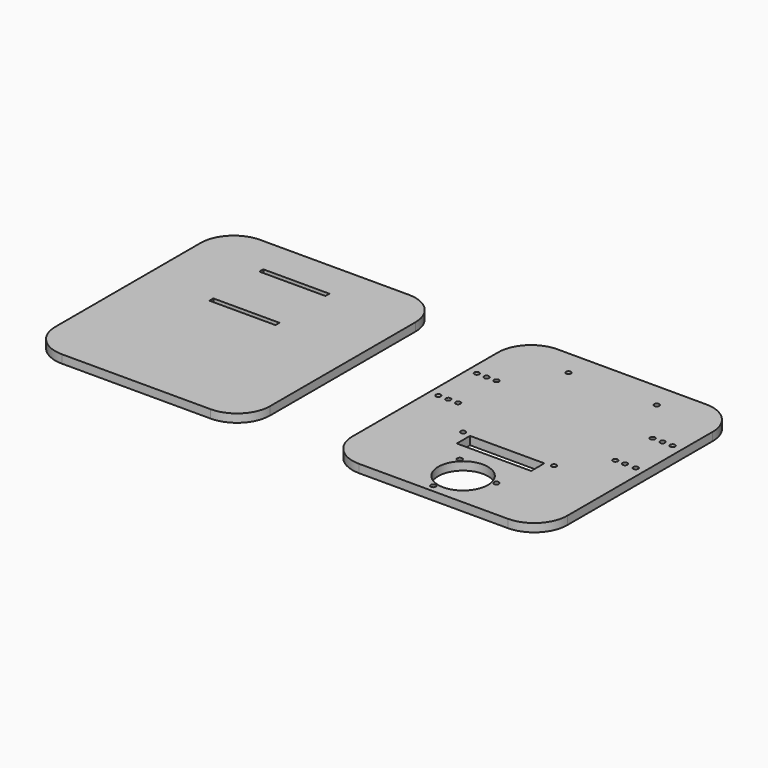
from build123d import *

# Parameters (mm, degrees)
F0_R     = 1.5000012089
F0_R_2   = 15.0000120892
F0_W     = 63
F0_H     = 28
F0_R_3   = 1.5
F0_W_2   = 45
F0_H_2   = 10
F1_DEPTH = 5
F0_W_3   = 40
F0_H_3   = 3
F2_DEPTH = 5


# Not quite as in the source:
# - a feature names something its author has since deleted; it is built from what else it names


with BuildPart() as f1:
    # F0 (on Top) → F1 (new body)
    with BuildSketch(Plane.XY):
        with BuildLine():
            Line((109.2777046029, -4.8284545538), (19.2777046029, -4.7197510892))
            ThreePointArc((19.2777046029, -4.7197510892), (5.1199557962, -10.5690629101), (-0.746451705, -24.719736501))
            Line((-0.746451705, -24.719736501), (-0.746451705, -134.8525817028))
            ThreePointArc((-0.746451705, -134.8525817028), (5.1114126713, -148.9947173266), (19.253548295, -154.8525817028))
            Line((19.253548295, -154.8525817028), (109.253548295, -154.8525817028))
            ThreePointArc((109.253548295, -154.8525817028), (123.3956839188, -148.9947173266), (129.253548295, -134.8525817028))
            Line((129.253548295, -134.8525817028), (129.253548295, -24.8284399656))
            ThreePointArc((129.253548295, -24.8284399656), (123.404221886, -10.6948474668), (109.2777046029, -4.8284545538))
        make_face()
        with Locations((60.6492295242, -150.5000877334)):
            Circle(F0_R, mode=Mode.SUBTRACT)
        with Locations((65.3296712528, -133.7744518814)):
            Circle(F0_R_2, mode=Mode.SUBTRACT)
        with Locations((82.2305977345, -129.661552608)):
            Circle(F0_R, mode=Mode.SUBTRACT)
        with Locations((53.3932128331, -121.3908070522)):
            Circle(F0_R, mode=Mode.SUBTRACT)
        with Locations((64.7868365049, -98.7337777073)):
            Rectangle(F0_W, F0_H, mode=Mode.SUBTRACT)
        with Locations((4.8244629152, -76.8351420979)):
            Circle(F0_R, mode=Mode.SUBTRACT)
        with Locations((10.8244677509, -76.8464319149)):
            Circle(F0_R, mode=Mode.SUBTRACT)
        with Locations((16.8244725865, -76.8634664953)):
            Circle(F0_R, mode=Mode.SUBTRACT)
        with Locations((4.8244629152, -47.7516189505)):
            Circle(F0_R, mode=Mode.SUBTRACT)
        with Locations((10.8244677509, -47.8464085426)):
            Circle(F0_R, mode=Mode.SUBTRACT)
        with Locations((16.8244725865, -47.8634431229)):
            Circle(F0_R, mode=Mode.SUBTRACT)
        with Locations((111.5633096981, -76.4066539684)):
            Circle(F0_R, mode=Mode.SUBTRACT)
        with Locations((117.3776644514, -76.3863511993)):
            Circle(F0_R, mode=Mode.SUBTRACT)
        with Locations((123.9776462317, -76.4066539684)):
            Circle(F0_R, mode=Mode.SUBTRACT)
        with Locations((111.2195700407, -47.7516189505)):
            Circle(F0_R, mode=Mode.SUBTRACT)
        with Locations((117.2429174185, -47.7516189505)):
            Circle(F0_R, mode=Mode.SUBTRACT)
        with Locations((123.3468130231, -47.7516189505)):
            Circle(F0_R, mode=Mode.SUBTRACT)
        with Locations((38.2347119981, -20.1513972986)):
            Circle(F0_R_3, mode=Mode.SUBTRACT)
        with Locations((91.4401854171, -19.9359528023)):
            Circle(F0_R_3, mode=Mode.SUBTRACT)
        with Locations((64.7868365049, -98.7337777073)):
            Rectangle(F0_W, F0_H)
        with Locations((37.2868365049, -98.7337777073)):
            Circle(F0_R_3, mode=Mode.SUBTRACT)
        with Locations((64.7868365049, -104.7337777073)):
            Rectangle(F0_W_2, F0_H_2, mode=Mode.SUBTRACT)
        with Locations((92.2868365049, -98.7337777073)):
            Circle(F0_R_3, mode=Mode.SUBTRACT)
    extrude(amount=F1_DEPTH)


with BuildPart() as f2:
    # F0 (on Top) → F2 (new body)
    with BuildSketch(Plane.XY):
        with BuildLine():
            Line((-70.49592942, -5.0235935599), (-160.49592942, -5.0235935599))
            ThreePointArc((-160.49592942, -5.0235935599), (-174.6380650437, -10.8814579361), (-180.49592942, -25.0235935599))
            Line((-180.49592942, -25.0235935599), (-180.49592942, -135.0235935599))
            ThreePointArc((-180.49592942, -135.0235935599), (-174.6380650437, -149.1657291836), (-160.49592942, -155.0235935599))
            Line((-160.49592942, -155.0235935599), (-70.49592942, -155.0235935599))
            ThreePointArc((-70.49592942, -155.0235935599), (-56.3537937963, -149.1657291836), (-50.49592942, -135.0235935599))
            Line((-50.49592942, -135.0235935599), (-50.49592942, -25.0235935599))
            ThreePointArc((-50.49592942, -25.0235935599), (-56.3537937963, -10.8814579361), (-70.49592942, -5.0235935599))
        make_face()
        with Locations((-120.3460991383, -67.1373978257)):
            Rectangle(F0_W_3, F0_H_3, mode=Mode.SUBTRACT)
        with Locations((-120.5274779797, -29.1373978257)):
            Rectangle(F0_W_3, F0_H_3, mode=Mode.SUBTRACT)
    extrude(amount=F2_DEPTH)


solid = Compound([f1.part, f2.part])
